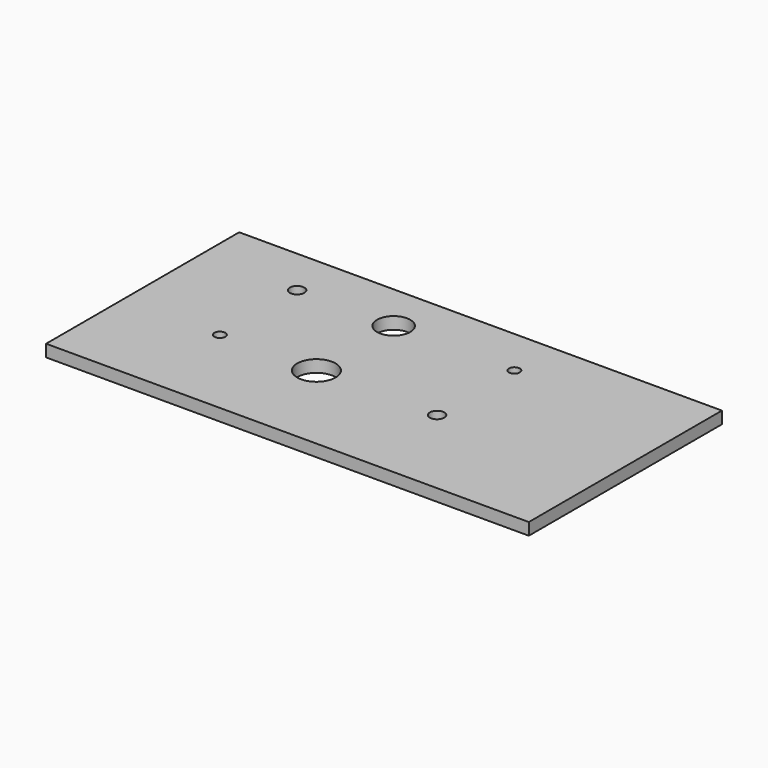
from build123d import *

# Parameters (mm, degrees)
F0_W     = 127
F0_H     = 63.5
F1_DEPTH = 3.175
F3_D     = 3.7973
F4_D     = 2.8702
F5_D     = 8.73125
F6_D     = 10.0838


# Not quite as in the source:
# - a length typed as a fraction of an inch, garbled in the dataset ("3 / 203.2 mm" for 3/8 in), is restored


with BuildPart() as f1:
    # F0 (on Top) → F1 (new body)
    with BuildSketch(Plane.XY):
        with Locations((63.5, 31.75)):
            Rectangle(F0_W, F0_H)
    extrude(amount=F1_DEPTH)

    # F3 (through all)
    with Locations(Plane.XY.offset(3.175)):
        with Locations((25.4, 50.8), (82.55, 25.4)):
            Hole(F3_D / 2)

    # F4 (through all)
    with Locations(Plane.XY.offset(3.175)):
        with Locations((25.4, 25.4), (82.55, 50.8)):
            Hole(F4_D / 2)

    # F5 (through all)
    with Locations(Plane.XY.offset(3.175)):
        with Locations((50.8, 50.8)):
            Hole(F5_D / 2)

    # F6 (through all)
    with Locations(Plane.XY.offset(3.175)):
        with Locations((50.8, 25.4)):
            Hole(F6_D / 2)


solid = f1.part
